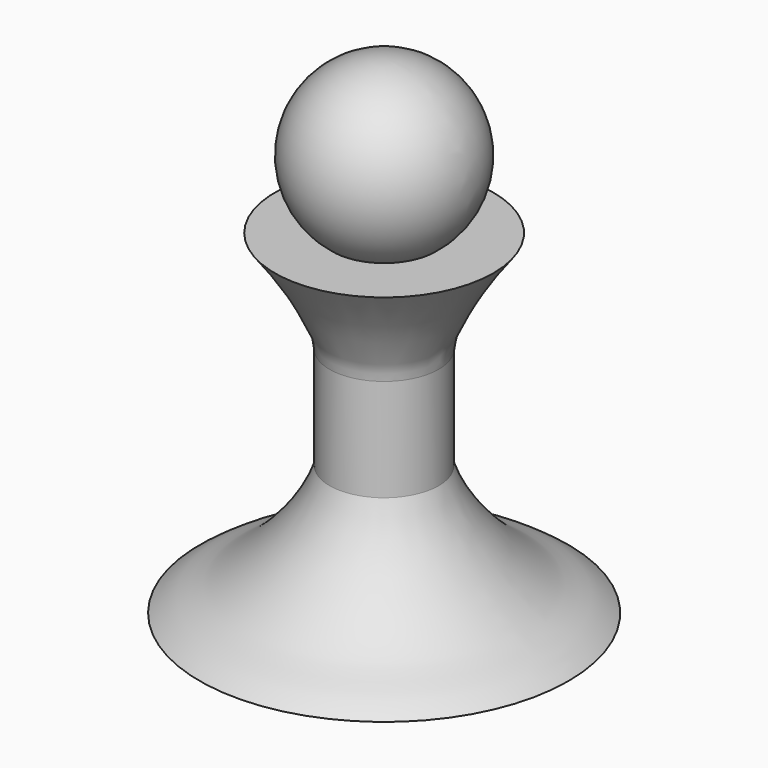
from build123d import *


with BuildPart() as f1:
    # F0 (on Front) → F1 (revolve)
    with BuildSketch(Plane.XZ):
        with BuildLine():
            Line((16, 17.0012365282), (7.5, 17.0012365282))
            ThreePointArc((7.5, 17.0012365282), (11.8585412256, 30.9540836034), (0, 39.5012365282))
            Line((0, 39.5012365282), (0, 27.0012365282))
            Line((0, 27.0012365282), (0, 17.0012365282))
            Line((0, 17.0012365282), (0, 2.0012365282))
            Line((0, 2.0012365282), (0, -12.9987634718))
            Line((0, -12.9987634718), (0, -27.9987634718))
            Line((0, -27.9987634718), (0, -29.9987634718))
            Line((0, -29.9987634718), (0, -31.9987634718))
            Line((0, -31.9987634718), (27, -31.9987634718))
            add(Edge.make_bspline(
                [(8, -12.9987634718), (10.1092817881, -19.655615647), (19.4790722356, -28.5878077637), (23.7774183733, -29.6020737173), (26.2356764407, -31.4218427093), (27, -31.9987634718)],
                knots=[0.6057411671, 0.6057411671, 0.6057411671, 0.6057411671, 0.8115404241, 0.9108393863, 1, 1, 1, 1], degree=3))
            add(Edge.make_bspline(
                [(8, 2.0012365282), (7.5604020354, -0.7405333825), (6.1360955685, -7.1163174472), (8, -12.9987634718)],
                knots=[0.4238829871, 0.4238829871, 0.4238829871, 0.4238829871, 0.6057411671, 0.6057411671, 0.6057411671, 0.6057411671], degree=3))
            add(Edge.make_bspline(
                [(16, 17.0012365282), (14.3141693383, 14.8802017595), (12.1375620782, 11.541444808), (10.8229786228, 9.300275817), (9.2727160233, 6.3116447724), (8.2168165295, 4.0954926116), (8.1681689979, 3.0501055757), (8, 2.0012365282)],
                knots=[0, 0, 0, 0, 0.1224696071, 0.1978563108, 0.283222856, 0.3543128108, 0.4238829871, 0.4238829871, 0.4238829871, 0.4238829871], degree=3))
        make_face()
        with BuildLine():
            Line((8, -12.9987634718), (8, 2.0012365282))
            add(Edge.make_bspline(
                [(8, 2.0012365282), (7.5604020354, -0.7405333825), (6.1360955685, -7.1163174472), (8, -12.9987634718)],
                knots=[0.4238829871, 0.4238829871, 0.4238829871, 0.4238829871, 0.6057411671, 0.6057411671, 0.6057411671, 0.6057411671], degree=3))
        make_face()
    revolve(axis=Axis((0, 0, 9.5012365282), (0, 0, -1)))


solid = f1.part
